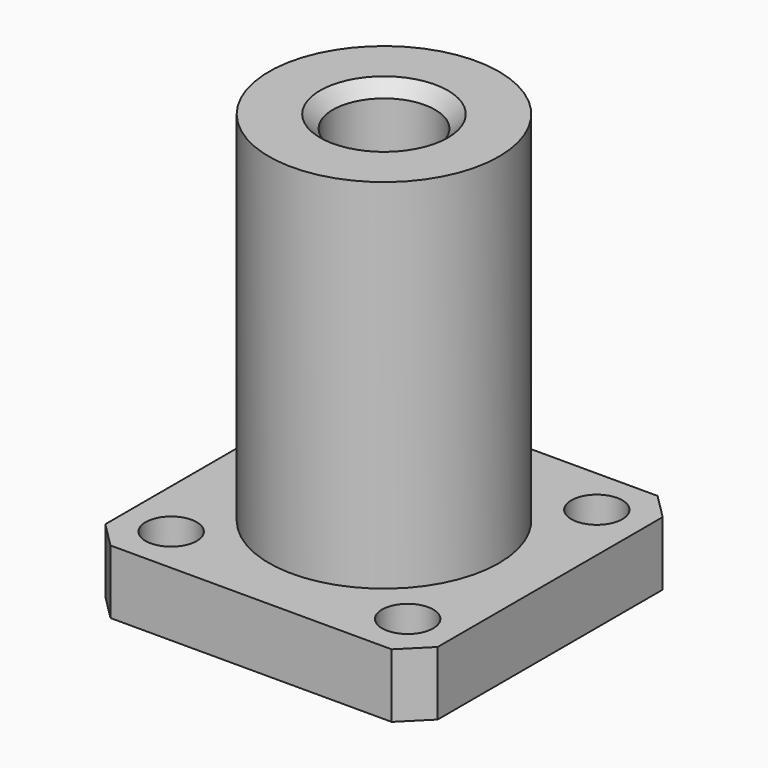
from build123d import *

# Parameters (mm, degrees)
F0_R      = 2.25
F0_R_2    = 1.5
F1_DEPTH  = 5.5
F2_W      = 0.5
F2_H      = 0.5
F4_R      = 3
F4_R_2    = 2
F5_DEPTH  = 7.5
F6_W      = 0.3
F6_H      = 0.5
F8_W      = 26
F8_H      = 26
F8_R      = 2
F8_R_2    = 4
F9_DEPTH  = 5
F10_R     = 9
F10_R_2   = 4
F11_DEPTH = 28
F12_SIZE  = 2
F13_SIZE  = 1
F14_R     = 5.75
F15_DEPTH = 1
F16_R     = 5
F17_DEPTH = 3
F18_R     = 1.5
F19_DEPTH = 4.001
F20_SIZE  = 0.25


with BuildPart() as f1:
    # F0 (on Top) → F1 (new body)
    with BuildSketch(Plane.XY):
        Circle(F0_R)
        Circle(F0_R_2, mode=Mode.SUBTRACT)
    extrude(amount=F1_DEPTH)

    # F2 (on Front) → F3 (revolve, cut)
    with BuildSketch(Plane.XZ):
        with Locations((2, 4.75)):
            Rectangle(F2_W, F2_H)
        Polygon((2.25, 4.1), (2.25, 4.5), (1.75, 4.1), align=None)
        Polygon((2.25, 3.7), (2.25, 4.1), (1.75, 3.7), align=None)
        Polygon((2.25, 3.3), (2.25, 3.7), (1.75, 3.3), align=None)
        Polygon((2.25, 2.9), (2.25, 3.3), (1.75, 2.9), align=None)
        Polygon((2.25, 2.5), (2.25, 2.9), (1.75, 2.5), align=None)
        Polygon((2.25, 2.1), (2.25, 2.5), (1.75, 2.1), align=None)
        Polygon((2.25, 1.7), (2.25, 2.1), (1.75, 1.7), align=None)
        Polygon((2.25, 1.3), (2.25, 1.7), (1.75, 1.3), align=None)
        Polygon((2.25, 0.6), (2.25, 1.3), (1.75, 0.9), (1.75, 0.6), align=None)
        Polygon((2.25, 0), (2.25, 0.3), (1.95, 0), align=None)
    revolve(axis=Axis((0, 0, 0), (0, 0, -1)), mode=Mode.SUBTRACT)


with BuildPart() as f5:
    # F4 (on Top) → F5 (new body)
    with BuildSketch(Plane.XY):
        Circle(F4_R)
        Circle(F4_R_2, mode=Mode.SUBTRACT)
    extrude(amount=F5_DEPTH)

    # F6 (on Front) → F7 (revolve, cut)
    with BuildSketch(Plane.XZ):
        with Locations((2.85, 6.75)):
            Rectangle(F6_W, F6_H)
        Polygon((3, 6.0615384615), (3, 6.5), (2.7, 6.0615384615), align=None)
        Polygon((3, 5.6230769231), (3, 6.0615384615), (2.7, 5.6230769231), align=None)
        Polygon((3, 5.1846153846), (3, 5.6230769231), (2.7, 5.1846153846), align=None)
        Polygon((3, 4.7461538462), (3, 5.1846153846), (2.7, 4.7461538462), align=None)
        Polygon((3, 4.3076923077), (3, 4.7461538462), (2.7, 4.3076923077), align=None)
        Polygon((3, 3.8692307692), (3, 4.3076923077), (2.7, 3.8692307692), align=None)
        Polygon((3, 3.4307692308), (3, 3.8692307692), (2.7, 3.4307692308), align=None)
        Polygon((3, 2.5538461538), (3, 2.9923076923), (2.7, 2.5538461538), align=None)
        Polygon((3, 2.9923076923), (3, 3.4307692308), (2.7, 2.9923076923), align=None)
        Polygon((3, 2.1153846154), (3, 2.5538461538), (2.7, 2.1153846154), align=None)
        Polygon((3, 1.6769230769), (3, 2.1153846154), (2.7, 1.6769230769), align=None)
        Polygon((3, 1.2384615385), (3, 1.6769230769), (2.7, 1.2384615385), align=None)
        Polygon((3, 0.5), (3, 1.2384615385), (2.7, 0.8), (2.7, 0.5), align=None)
        Polygon((3, 0), (3, 0.3), (2.7, 0), align=None)
    revolve(axis=Axis((0, 0, 0), (0, 0, -1)), mode=Mode.SUBTRACT)


with BuildPart() as f9:
    # F8 (on Top) → F9 (new body)
    with BuildSketch(Plane.XY):
        Rectangle(F8_W, F8_H)
        with Locations((-9.25, -9.25)):
            Circle(F8_R, mode=Mode.SUBTRACT)
        with Locations((9.25, -9.25)):
            Circle(F8_R, mode=Mode.SUBTRACT)
        with Locations((-9.25, 9.25)):
            Circle(F8_R, mode=Mode.SUBTRACT)
        Circle(F8_R_2, mode=Mode.SUBTRACT)
        with Locations((9.25, 9.25)):
            Circle(F8_R, mode=Mode.SUBTRACT)
    extrude(amount=F9_DEPTH)

    # F10 (on face) → F11 (join)
    with BuildSketch(Plane.XY.offset(5)):
        Circle(F10_R)
        Circle(F10_R_2, mode=Mode.SUBTRACT)
    extrude(amount=F11_DEPTH)

    # F12
    f12_edges = [f9.edges().sort_by_distance(p)[0] for p in [
        (-13, -13, 2.5),
        (13, -13, 2.5),
        (13, 13, 2.5),
        (-13, 13, 2.5),
    ]]
    chamfer(f12_edges, length=F12_SIZE)

    # F13
    f13_edges = [f9.edges().sort_by_distance(p)[0] for p in [
        (-4, 0, 33),
        (-4, 0, 0),
    ]]
    chamfer(f13_edges, length=F13_SIZE)


with BuildPart() as f15:
    # F14 (on Top) → F15 (new body)
    with BuildSketch(Plane.XY):
        Circle(F14_R)
    extrude(amount=F15_DEPTH)

    # F16 (on face) → F17 (join)
    with BuildSketch(Plane.XY.offset(1)):
        Circle(F16_R)
    extrude(amount=F17_DEPTH)

    # F18 (on face) → F19 (cut, through all)
    with BuildSketch(Plane.XY.offset(4)):
        Circle(F18_R)
    extrude(amount=-F19_DEPTH, mode=Mode.SUBTRACT)

    # F20
    f20_edges = [f15.edges().sort_by_distance(p)[0] for p in [
        (-5, 0, 4),
        (-1.5, 0, 4),
        (-5.75, 0, 1),
        (-5.75, 0, 0),
        (-1.5, 0, 0),
    ]]
    chamfer(f20_edges, length=F20_SIZE)


solid = Compound([f1.part, f5.part, f9.part, f15.part])
